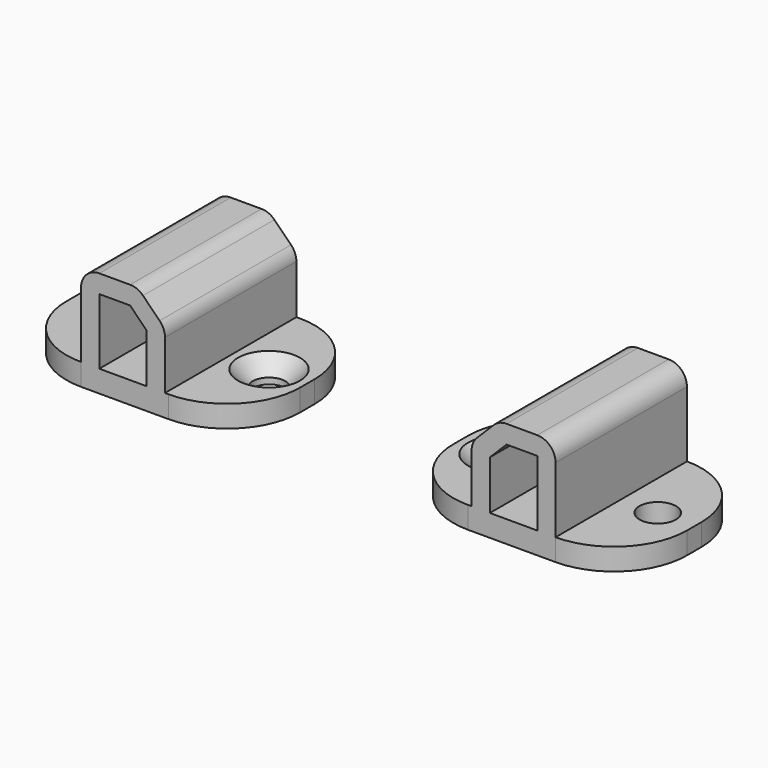
from build123d import *

# Parameters (mm, degrees)
F6_DEPTH        = 5
F7_DEPTH        = 20
F8_DEPTH        = 40
F9_DEPTH        = 25
F10_R           = 5
F11_R           = 20
F12_D           = 9
F12_DEPTH       = 8
F12_CSINK_D     = 17
F12_CSINK_ANGLE = 85.294
F12_TIP         = 2.7038727856
F13_D           = 10
F13_DEPTH       = 8
F13_TIP         = 3.0043030951


# Not quite as in the source:
# - a feature names something its author has since deleted; it is built from what else it names


with BuildPart() as f6:
    # F3 (on Front) → F6 (new body)
    with BuildSketch(Plane.XZ):
        Polygon((-44, 0), (0, 0), (20, 0), (20, 6), (-44, 6), align=None)
    extrude(amount=F6_DEPTH)

    # F4 (on offset) → F7 (join)
    with BuildSketch(Plane.XZ.offset(-15)):
        Polygon((-5, 6), (0, 6), (0, 29), (-15.5, 29), (-23, 21.5), (-23, 6), (-18, 6), (-18, 19.4289321881), (-13.4289321881, 24), (-5, 24), align=None)
    extrude(amount=F7_DEPTH)

    # F3 (on Front) → F8 (join)
    with BuildSketch(Plane.XZ):
        Polygon((-44, 0), (0, 0), (20, 0), (20, 6), (-44, 6), align=None)
    extrude(amount=-F8_DEPTH)

    # F4 (on offset) → F9 (join)
    with BuildSketch(Plane.XZ.offset(-15)):
        Polygon((-5, 6), (0, 6), (0, 29), (-15.5, 29), (-23, 21.5), (-23, 6), (-18, 6), (-18, 19.4289321881), (-13.4289321881, 24), (-5, 24), align=None)
    extrude(amount=-F9_DEPTH)

    # F10
    f10_edges = [f6.edges().sort_by_distance(p)[0] for p in [
        (-15.5, 17.5, 29),
        (-23, 17.5, 21.5),
        (0, 17.5, 29),
    ]]
    fillet(f10_edges, radius=F10_R)

    # F11
    f11_edges = [f6.edges().sort_by_distance(p)[0] for p in [
        (20, -5, 3),
        (20, 40, 3),
        (-44, 40, 3),
        (-44, -5, 3),
    ]]
    fillet(f11_edges, radius=F11_R)

    # F12
    with Locations(Plane.XY.offset(6)):
        with Locations((-33.5, 17.5)):
            CounterSinkHole(F12_D / 2, F12_CSINK_D / 2, depth=F12_DEPTH, counter_sink_angle=F12_CSINK_ANGLE)
            with Locations((0, 0, -(F12_DEPTH + F12_TIP / 2))):  # 118° drill point
                Cone(0, F12_D / 2, F12_TIP, mode=Mode.SUBTRACT)

    # F13
    with Locations(Plane.XY.offset(6)):
        with Locations((10, 17.5)):
            Hole(F13_D / 2, depth=F13_DEPTH)
            with Locations((0, 0, -(F13_DEPTH + F13_TIP / 2))):  # 118° drill point
                Cone(0, F13_D / 2, F13_TIP, mode=Mode.SUBTRACT)


with BuildPart() as f15_1:
    # F15: instance of F6
    add(f6.part.mirror(Plane.YZ.offset(-65)))


solid = Compound([f6.part, f15_1.part])
